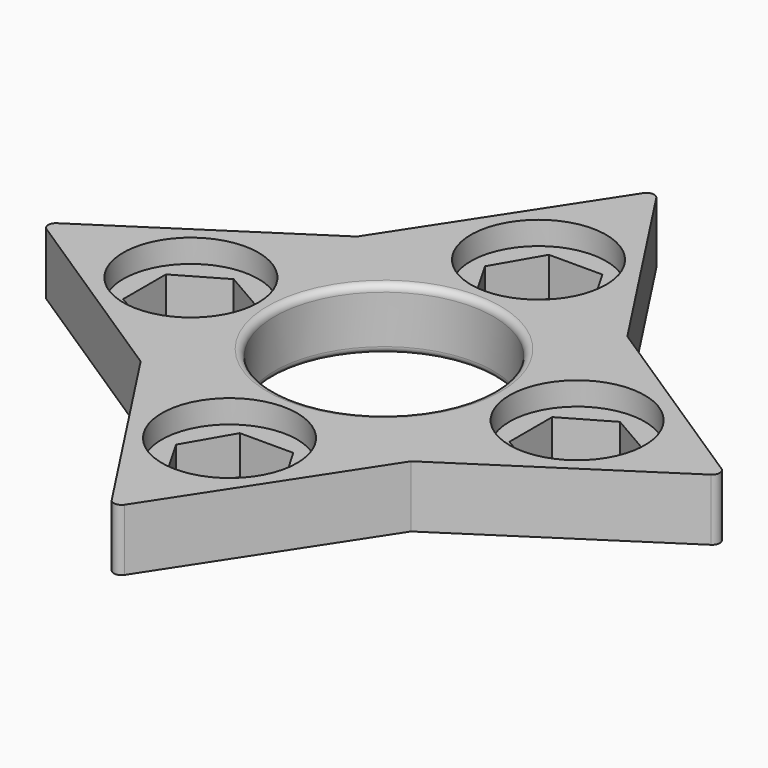
from build123d import *

# Parameters (mm, degrees)
F0_W            = 35
F0_H            = 35
F0_R            = 14.15
F1_DEPTH        = 8
F3_DEPTH        = 25
F3_COPIES_COUNT = 3
F3_COPIES_ANGLE = 180
F4_R            = 8.75
F5_DEPTH        = 3
F5_COPIES_COUNT = 3
F5_COPIES_ANGLE = 180
F7_DEPTH        = 25
F8_R            = 8.75
F9_DEPTH        = 3
F10_R           = 1
F11_R           = 0.9


# Not quite as in the source:
# - a pattern or mirror of a feature is missing from the dataset's text; its kind, count and spacing are read off the source's solid


with BuildPart() as f1:
    # F0 (on Top) → F1 (new body)
    with BuildSketch(Plane.XY):
        Polygon((0, -44.2908566492), (17.5, -17.5), (-17.5, -17.5), align=None)
        Polygon((17.5, 17.5), (17.5, -17.5), (44.2908566492, 0), align=None)
        Polygon((-44.2908566492, 0), (-17.5, -17.5), (-17.5, 17.5), align=None)
        Rectangle(F0_W, F0_H)
        Circle(F0_R, mode=Mode.SUBTRACT)
        Polygon((-17.5, 17.5), (17.5, 17.5), (0, 44.2908566492), align=None)
    extrude(amount=F1_DEPTH)

    # F2 (on face) → F3 (cut)
    with BuildSketch(Plane.XY.offset(8)):
        Polygon((-19, -3.4641016151), (-19, 3.4641016151), (-25, 6.9282032303), (-31, 3.4641016151), (-31, -3.4641016151), (-25, -6.9282032303), align=None)
    f3 = extrude(amount=-F3_DEPTH, mode=Mode.SUBTRACT)

    # F3_copies: F3 ×3 about axis
    f3_copies_axis = Axis((0, 0, 0), (0, 0, -1))
    for i in range(1, F3_COPIES_COUNT):
        add(f3.rotate(f3_copies_axis, i * F3_COPIES_ANGLE / (F3_COPIES_COUNT - 1)), mode=Mode.SUBTRACT)

    # F4 (on face) → F5 (cut)
    with BuildSketch(Plane.XY.offset(8)):
        with Locations((-25, 0)):
            Circle(F4_R)
        Polygon((-19, 3.4641016151), (-19, -3.4641016151), (-25, -6.9282032303), (-31, -3.4641016151), (-31, 3.4641016151), (-25, 6.9282032303), align=None, mode=Mode.SUBTRACT)
    f5 = extrude(amount=-F5_DEPTH, mode=Mode.SUBTRACT)

    # F5_copies: F5 ×3 about axis
    f5_copies_axis = Axis((0, 0, 0), (0, 0, -1))
    for i in range(1, F5_COPIES_COUNT):
        add(f5.rotate(f5_copies_axis, i * F5_COPIES_ANGLE / (F5_COPIES_COUNT - 1)), mode=Mode.SUBTRACT)

    # F6 (on face) → F7 (cut)
    with BuildSketch(Plane.XY.offset(8)):
        Polygon((3.4641016151, -19), (-3.4641016151, -19), (-6.9282032303, -25), (-3.4641016151, -31), (3.4641016151, -31), (6.9282032303, -25), align=None)
    extrude(amount=-F7_DEPTH, mode=Mode.SUBTRACT)

    # F8 (on face) → F9 (cut)
    with BuildSketch(Plane.XY.offset(8)):
        with Locations((0, -25)):
            Circle(F8_R)
        Polygon((-3.4641016151, -19), (3.4641016151, -19), (6.9282032303, -25), (3.4641016151, -31), (-3.4641016151, -31), (-6.9282032303, -25), align=None, mode=Mode.SUBTRACT)
    extrude(amount=-F9_DEPTH, mode=Mode.SUBTRACT)

    # F10
    f10_edges = [f1.edges().sort_by_distance(p)[0] for p in [
        (-44.290857, 0, 4),
        (0, 44.290857, 4),
        (0, -44.290857, 4),
        (44.290857, 0, 4),
    ]]
    fillet(f10_edges, radius=F10_R)

    # F11
    f11_edges = [f1.edges().sort_by_distance(p)[0] for p in [
        (-14.15, 0, 8),
        (-14.15, 0, 0),
    ]]
    fillet(f11_edges, radius=F11_R)


solid = f1.part
